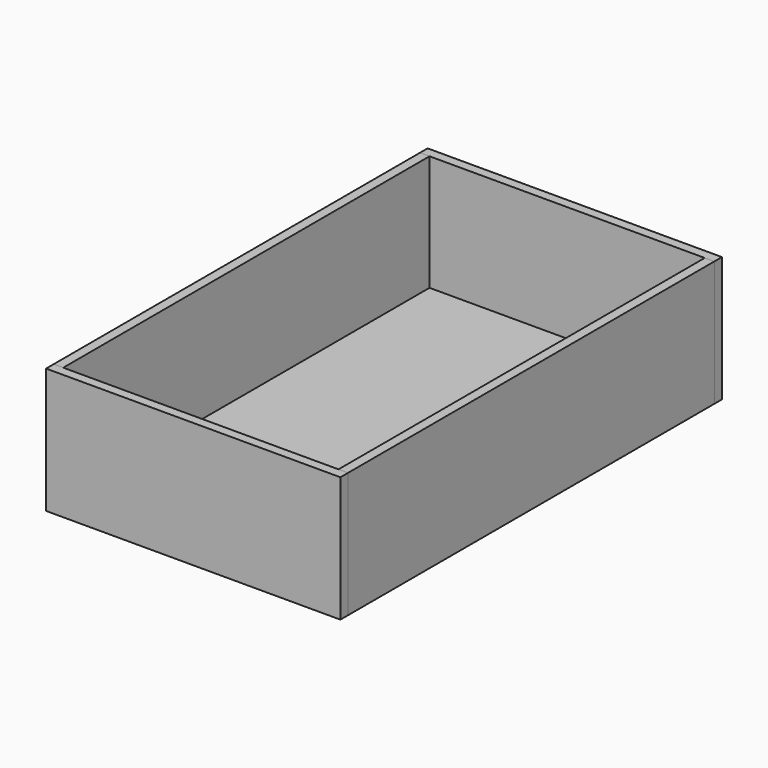
from build123d import *

# Parameters (mm, degrees)
F1_W     = 685.8
F1_H     = 292.1
F2_DEPTH = 22.225
F3_W     = 641.35
F3_H     = 1066.8
F4_DEPTH = 22.225
F5_W     = 1066.8
F5_H     = 292.1
F6_DEPTH = 22.225


# Not quite as in the source:
# - a variable given as a bare number and used for a length is read in inches; the dataset says mm whatever the document's units were
# - a length typed as a fraction of an inch, garbled in the dataset ("3 / 203.2 mm" for 3/8 in), is restored


with BuildPart() as f2:
    # F1 (on Front) → F2 (new body)
    with BuildSketch(Plane.XZ):
        with Locations((0, 146.05)):
            Rectangle(F1_W, F1_H)
    extrude(amount=-F2_DEPTH)


with BuildPart() as f4:
    # F3 (on face) → F4 (new body)
    with BuildSketch(Plane(origin=(0, 0, 0), x_dir=(1, 0, 0), z_dir=(0, 0, -1))):
        with Locations((0, -555.625)):
            Rectangle(F3_W, F3_H)
    extrude(amount=-F4_DEPTH)


with BuildPart() as f6:
    # F5 (on face) → F6 (new body)
    with BuildSketch(Plane.YZ.offset(342.9)):
        with Locations((555.625, 146.05)):
            Rectangle(F5_W, F5_H)
    extrude(amount=-F6_DEPTH)


with BuildPart() as f7_1:
    # F7: instance of F6
    add(f6.part.mirror(Plane.YZ))


with BuildPart() as f9_1:
    # F9: instance of F2
    add(f2.part.mirror(Plane(origin=(331.7875, 555.625, 146.05), x_dir=(1, 0, 0), z_dir=(0, -1, 0))))


solid = Compound([f2.part, f4.part, f6.part, f7_1.part, f9_1.part])
